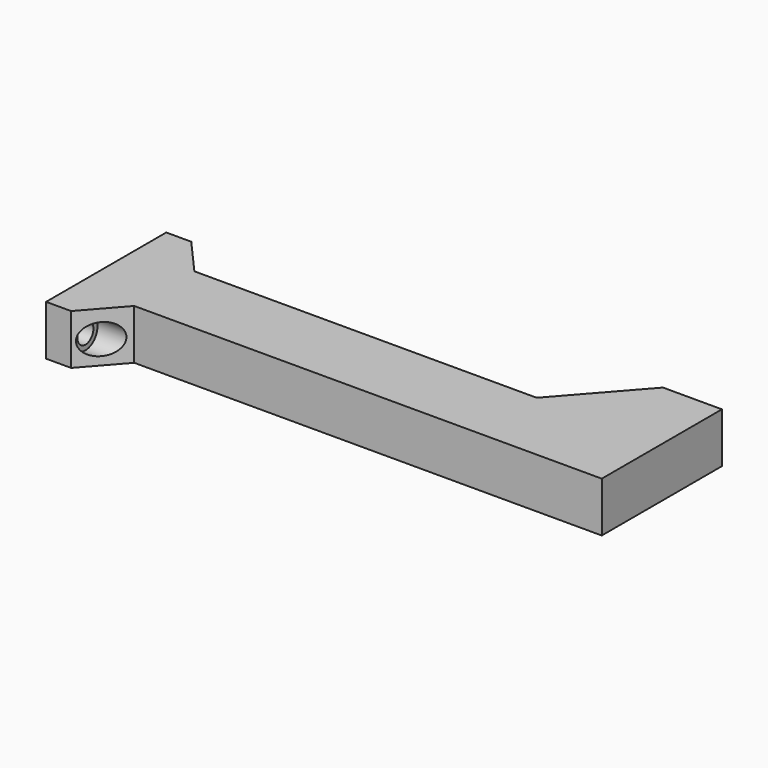
from build123d import *

# Parameters (mm, degrees)
F1_DEPTH  = 12.7
F2_W      = 9.525
F2_H      = 12.7
F2_R      = 2.54
F2_W_2    = 19.05
F3_DEPTH  = 6.35
F4_DEPTH  = 25.4
F6_DEPTH  = 12.7
F7_DEPTH  = 12.7
F8_R      = 3.8109417559
F8_R_2    = 2.54
F9_DEPTH  = 25.4
F10_R     = 3.81
F10_R_2   = 2.54
F11_DEPTH = 25.4


with BuildPart() as f1:
    # F0 (on Top) → F1 (new body)
    with BuildSketch(Plane.XY):
        Polygon((63.5, 19.05), (48.5505208253, 19.05), (31.75, 0), (-63.5, 0), (-63.5, -19.05), (63.5, -19.05), align=None)
    extrude(amount=F1_DEPTH)

    # F2 (on face) → F3 (join)
    with BuildSketch(Plane(origin=(-63.5, 0, 0), x_dir=(0, -1, 0), z_dir=(-1, 0, 0))):
        with Locations((-4.7625, 6.35)):
            Rectangle(F2_W, F2_H)
        with Locations((-5.3587416187, 5.8867353946)):
            Circle(F2_R, mode=Mode.SUBTRACT)
        with Locations((9.525, 6.35)):
            Rectangle(F2_W_2, F2_H)
        with Locations((23.8125, 6.35)):
            Rectangle(F2_W, F2_H)
        with Locations((24.0348111838, 5.8867353946)):
            Circle(F2_R, mode=Mode.SUBTRACT)
    extrude(amount=F3_DEPTH)

    # F2 (on face) → F4 (cut)
    with BuildSketch(Plane(origin=(-63.5, 0, 0), x_dir=(0, -1, 0), z_dir=(-1, 0, 0))):
        with Locations((24.0348111838, 5.8867353946)):
            Circle(F2_R)
    extrude(amount=F4_DEPTH, mode=Mode.SUBTRACT)

    # F5 (on face) → F6 (join)
    with BuildSketch(Plane.XY.offset(12.7)):
        Polygon((-55.0928376615, 0), (-63.5, 9.525), (-63.5, 0), align=None)
    extrude(amount=-F6_DEPTH)

    # F5 (on face) → F7 (join)
    with BuildSketch(Plane.XY.offset(12.7)):
        Polygon((-63.5, -19.05), (-63.5, -28.575), (-55.1101081073, -19.05), align=None)
    extrude(amount=-F7_DEPTH)

    # F8 (on face) → F9 (cut)
    with BuildSketch(Plane(origin=(-63.5, 0, 0), x_dir=(0, -1, 0), z_dir=(-1, 0, 0))):
        with Locations((-5.3587416187, 5.8867353946)):
            Circle(F8_R)
        with Locations((-5.3587416187, 5.8867353946)):
            Circle(F8_R_2, mode=Mode.SUBTRACT)
        with Locations((-5.3587416187, 5.8867353946)):
            Circle(F8_R_2)
    extrude(amount=-F9_DEPTH, mode=Mode.SUBTRACT)

    # F10 (on face) → F11 (cut)
    with BuildSketch(Plane(origin=(-63.5, 0, 0), x_dir=(0, -1, 0), z_dir=(-1, 0, 0))):
        with Locations((24.0348111838, 5.8867353946)):
            Circle(F10_R)
        with Locations((24.0348111838, 5.8867353946)):
            Circle(F10_R_2, mode=Mode.SUBTRACT)
        with Locations((24.0348111838, 5.8867353946)):
            Circle(F10_R_2)
    extrude(amount=-F11_DEPTH, mode=Mode.SUBTRACT)


solid = f1.part
